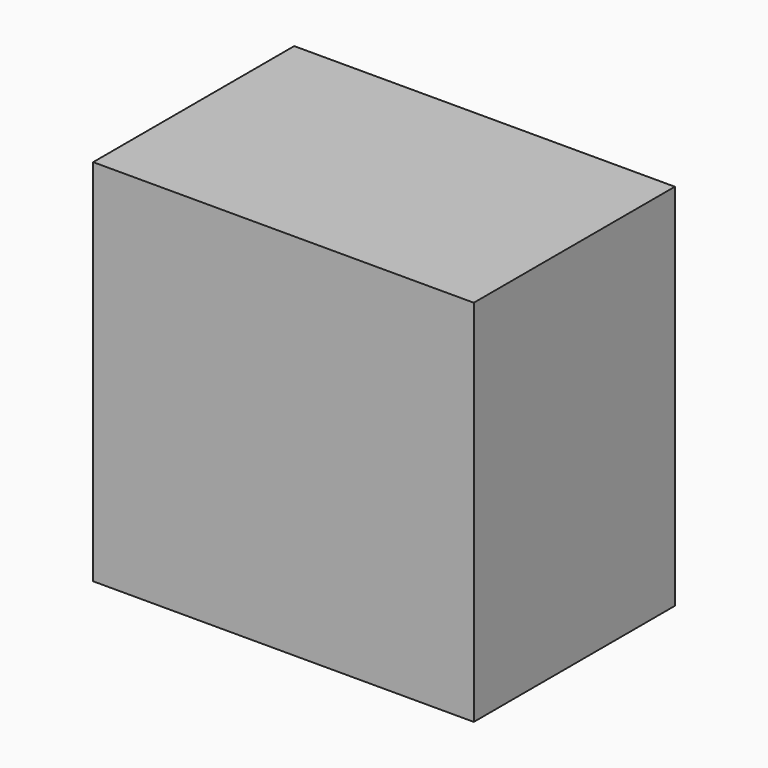
from build123d import *

# Parameters (mm, degrees)
F0_W     = 37.8679335117
F0_H     = 36.7116522975
F1_DEPTH = 25


with BuildPart() as f1:
    # F0 (on Front) → F1 (new body)
    with BuildSketch(Plane.XZ):
        with Locations((-223.4496772289, 23.125452688)):
            Rectangle(F0_W, F0_H)
    extrude(amount=F1_DEPTH)


solid = f1.part
